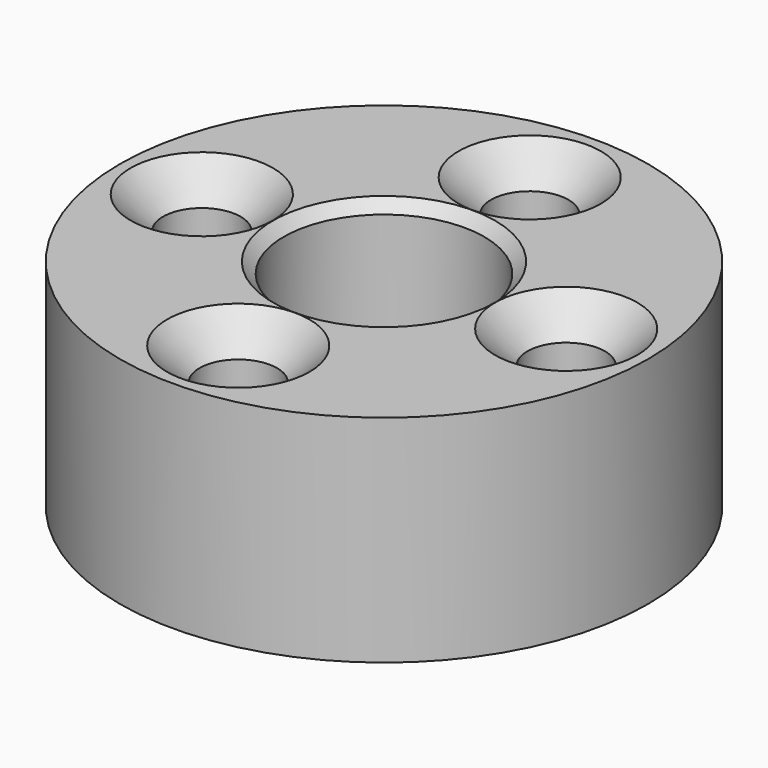
from build123d import *

# Parameters (mm, degrees)
F0_R     = 12.25
F0_R_2   = 1.8
F0_R_3   = 4.65
F1_DEPTH = 10
F2_SIZE  = 1.5
F3_SIZE  = 0.49999


# Not quite as in the source:
# - a fillet or chamfer is up to 0.001 mm smaller than in the source, because OpenCascade refuses the exact size


with BuildPart() as f1:
    # F0 (on Top) → F1 (new body)
    with BuildSketch(Plane.XY):
        Circle(F0_R)
        with Locations((0, -8.45)):
            Circle(F0_R_2, mode=Mode.SUBTRACT)
        with Locations((-8.45, 0)):
            Circle(F0_R_2, mode=Mode.SUBTRACT)
        Circle(F0_R_3, mode=Mode.SUBTRACT)
        with Locations((8.45, 0)):
            Circle(F0_R_2, mode=Mode.SUBTRACT)
        with Locations((0, 8.45)):
            Circle(F0_R_2, mode=Mode.SUBTRACT)
    extrude(amount=F1_DEPTH)

    # F2
    f2_edges = [f1.edges().sort_by_distance(p)[0] for p in [
        (-10.25, 0, 10),
        (-1.8, 8.45, 10),
        (6.65, 0, 10),
        (-1.8, -8.45, 10),
    ]]
    chamfer(f2_edges, length=F2_SIZE)

    # F3 (size 0.5 in the source; OpenCascade refuses exactly that, so slightly less here)
    f3_edges = [f1.edges().sort_by_distance(p)[0] for p in [
        (-4.65, 0, 10),
    ]]
    chamfer(f3_edges, length=F3_SIZE)


solid = f1.part
